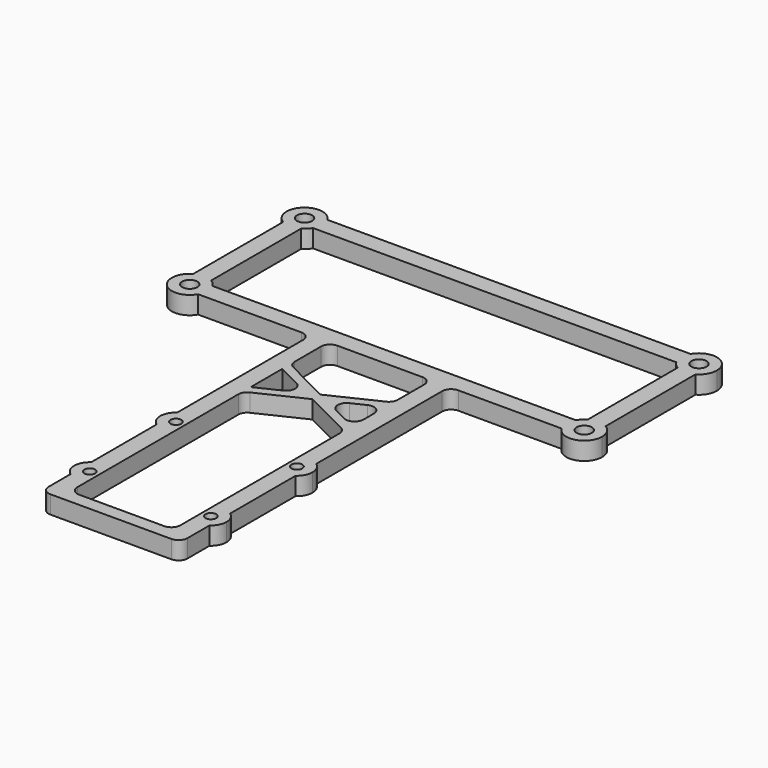
from build123d import *

# Parameters (mm, degrees)
F0_R     = 0.6
F0_R_2   = 0.85
F1_DEPTH = 2
F2_R     = 1


# Not quite as in the source:
# - a feature names something its author has since deleted; it is built from what else it names


with BuildPart() as f1:
    # F0 (on Top) → F1 (new body)
    with BuildSketch(Plane.XY):
        with BuildLine():
            ThreePointArc((-5.75, -27.5638593384), (-6.75, -27.25), (-7.75, -27.5638593384))
            Line((-7.75, -27.5638593384), (-7.75, -30.4361406616))
            ThreePointArc((-7.75, -30.4361406616), (-6.75, -30.75), (-5.75, -30.4361406616))
            Line((-5.75, -30.4361406616), (-5.75, -27.5638593384))
        make_face()
        with Locations((-6.75, -29)):
            Circle(F0_R, mode=Mode.SUBTRACT)
        with BuildLine():
            Line((-7.75, -30.4361406616), (-7.75, -27.5638593384))
            ThreePointArc((-7.75, -27.5638593384), (-8.5, -29), (-7.75, -30.4361406616))
        make_face()
        with BuildLine():
            ThreePointArc((-5.75, -30.4361406616), (-6.75, -30.75), (-7.75, -30.4361406616))
            Line((-7.75, -30.4361406616), (-7.75, -39.5638593384))
            ThreePointArc((-7.75, -39.5638593384), (-6.75, -39.25), (-5.75, -39.5638593384))
            Line((-5.75, -39.5638593384), (-5.75, -30.4361406616))
        make_face()
        with BuildLine():
            Line((-7.75, -42.4361406616), (-7.75, -39.5638593384))
            ThreePointArc((-7.75, -39.5638593384), (-8.5, -41), (-7.75, -42.4361406616))
        make_face()
        with BuildLine():
            ThreePointArc((-5.75, -39.5638593384), (-6.75, -39.25), (-7.75, -39.5638593384))
            Line((-7.75, -39.5638593384), (-7.75, -42.4361406616))
            ThreePointArc((-7.75, -42.4361406616), (-6.75, -42.75), (-5.75, -42.4361406616))
            Line((-5.75, -42.4361406616), (-5.75, -39.5638593384))
        make_face()
        with Locations((-6.75, -41)):
            Circle(F0_R, mode=Mode.SUBTRACT)
        with BuildLine():
            ThreePointArc((-5.75, -42.4361406616), (-6.75, -42.75), (-7.75, -42.4361406616))
            Line((-7.75, -42.4361406616), (-7.75, -46.5))
            Line((-7.75, -46.5), (7.75, -46.5))
            Line((7.75, -46.5), (7.75, -42.4361406616))
            ThreePointArc((7.75, -42.4361406616), (6.75, -42.75), (5.75, -42.4361406616))
            Line((5.75, -42.4361406616), (5.75, -45))
            Line((5.75, -45), (-5.75, -45))
            Line((-5.75, -45), (-5.75, -42.4361406616))
        make_face()
        with BuildLine():
            Line((7.75, -30.4361406616), (7.75, -27.5638593384))
            ThreePointArc((7.75, -27.5638593384), (6.75, -27.25), (5.75, -27.5638593384))
            Line((5.75, -27.5638593384), (5.75, -30.4361406616))
            ThreePointArc((5.75, -30.4361406616), (6.75, -30.75), (7.75, -30.4361406616))
        make_face()
        with Locations((6.75, -29)):
            Circle(F0_R, mode=Mode.SUBTRACT)
        with BuildLine():
            ThreePointArc((8.5, -29), (8.3012092057, -28.1899074127), (7.75, -27.5638593384))
            Line((7.75, -27.5638593384), (7.75, -30.4361406616))
            ThreePointArc((7.75, -30.4361406616), (8.3012092057, -29.8100925873), (8.5, -29))
        make_face()
        with BuildLine():
            Line((7.75, -39.5638593384), (7.75, -30.4361406616))
            ThreePointArc((7.75, -30.4361406616), (6.75, -30.75), (5.75, -30.4361406616))
            Line((5.75, -30.4361406616), (5.75, -39.5638593384))
            ThreePointArc((5.75, -39.5638593384), (6.75, -39.25), (7.75, -39.5638593384))
        make_face()
        with BuildLine():
            Line((7.75, -42.4361406616), (7.75, -39.5638593384))
            ThreePointArc((7.75, -39.5638593384), (6.75, -39.25), (5.75, -39.5638593384))
            Line((5.75, -39.5638593384), (5.75, -42.4361406616))
            ThreePointArc((5.75, -42.4361406616), (6.75, -42.75), (7.75, -42.4361406616))
        make_face()
        with Locations((6.75, -41)):
            Circle(F0_R, mode=Mode.SUBTRACT)
        with BuildLine():
            ThreePointArc((8.5, -41), (8.3012092057, -40.1899074127), (7.75, -39.5638593384))
            Line((7.75, -39.5638593384), (7.75, -42.4361406616))
            ThreePointArc((7.75, -42.4361406616), (8.3012092057, -41.8100925873), (8.5, -41))
        make_face()
        with BuildLine():
            ThreePointArc((-20, -8), (-20.0681483474, -8.5176380902), (-20.2679491924, -9))
            Line((-20.2679491924, -9), (-7.75, -9))
            Line((-7.75, -9), (-5.75, -9))
            Line((-5.75, -9), (5.75, -9))
            Line((5.75, -9), (7.75, -9))
            Line((7.75, -9), (20.2679491924, -9))
            ThreePointArc((20.2679491924, -9), (20, -8), (20.2679491924, -7))
            Line((20.2679491924, -7), (-20.2679491924, -7))
            ThreePointArc((-20.2679491924, -7), (-20.0681483474, -7.4823619098), (-20, -8))
        make_face()
        with BuildLine():
            ThreePointArc((24, -8), (23.7320508076, -7), (23, -6.2679491924))
            Line((23, -6.2679491924), (23, -9))
            Line((23, -9), (20.2679491924, -9))
            ThreePointArc((20.2679491924, -9), (22.5176380902, -9.9318516526), (24, -8))
        make_face()
        with BuildLine():
            ThreePointArc((23, -6.2679491924), (22, -6), (21, -6.2679491924))
            Line((21, -6.2679491924), (21, -7))
            Line((21, -7), (20.2679491924, -7))
            ThreePointArc((20.2679491924, -7), (20, -8), (20.2679491924, -9))
            Line((20.2679491924, -9), (23, -9))
            Line((23, -9), (23, -6.2679491924))
        make_face()
        with Locations((22, -8)):
            Circle(F0_R_2, mode=Mode.SUBTRACT)
        with BuildLine():
            ThreePointArc((23, 6.2679491924), (22, 6), (21, 6.2679491924))
            Line((21, 6.2679491924), (21, -6.2679491924))
            ThreePointArc((21, -6.2679491924), (22, -6), (23, -6.2679491924))
            Line((23, -6.2679491924), (23, 6.2679491924))
        make_face()
        with BuildLine():
            Line((21, -7), (21, -6.2679491924))
            ThreePointArc((21, -6.2679491924), (20.5857864376, -6.5857864376), (20.2679491924, -7))
            Line((20.2679491924, -7), (21, -7))
        make_face()
        with BuildLine():
            Line((21, 7), (20.2679491924, 7))
            ThreePointArc((20.2679491924, 7), (20.5857864376, 6.5857864376), (21, 6.2679491924))
            Line((21, 6.2679491924), (21, 7))
        make_face()
        with BuildLine():
            Line((23, 9), (20.2679491924, 9))
            ThreePointArc((20.2679491924, 9), (20, 8), (20.2679491924, 7))
            Line((20.2679491924, 7), (21, 7))
            Line((21, 7), (21, 6.2679491924))
            ThreePointArc((21, 6.2679491924), (22, 6), (23, 6.2679491924))
            Line((23, 6.2679491924), (23, 9))
        make_face()
        with Locations((22, 8)):
            Circle(F0_R_2, mode=Mode.SUBTRACT)
        with BuildLine():
            ThreePointArc((24, 8), (22.5176380902, 9.9318516526), (20.2679491924, 9))
            Line((20.2679491924, 9), (23, 9))
            Line((23, 9), (23, 6.2679491924))
            ThreePointArc((23, 6.2679491924), (23.7320508076, 7), (24, 8))
        make_face()
        with BuildLine():
            ThreePointArc((-20.2679491924, 9), (-20.0681483474, 8.5176380902), (-20, 8))
            ThreePointArc((-20, 8), (-20.0681483474, 7.4823619098), (-20.2679491924, 7))
            Line((-20.2679491924, 7), (20.2679491924, 7))
            ThreePointArc((20.2679491924, 7), (20, 8), (20.2679491924, 9))
            Line((20.2679491924, 9), (-20.2679491924, 9))
        make_face()
        with BuildLine():
            ThreePointArc((-21, -6.2679491924), (-22, -6), (-23, -6.2679491924))
            Line((-23, -6.2679491924), (-23, -9))
            Line((-23, -9), (-20.2679491924, -9))
            ThreePointArc((-20.2679491924, -9), (-20.0681483474, -8.5176380902), (-20, -8))
            ThreePointArc((-20, -8), (-20.0681483474, -7.4823619098), (-20.2679491924, -7))
            Line((-20.2679491924, -7), (-21, -7))
            Line((-21, -7), (-21, -6.2679491924))
        make_face()
        with Locations((-22, -8)):
            Circle(F0_R_2, mode=Mode.SUBTRACT)
        with BuildLine():
            Line((-23, -9), (-23, -6.2679491924))
            ThreePointArc((-23, -6.2679491924), (-23.4142135624, -9.4142135624), (-20.2679491924, -9))
            Line((-20.2679491924, -9), (-23, -9))
        make_face()
        with BuildLine():
            ThreePointArc((-20.2679491924, -7), (-20.5857864376, -6.5857864376), (-21, -6.2679491924))
            Line((-21, -6.2679491924), (-21, -7))
            Line((-21, -7), (-20.2679491924, -7))
        make_face()
        with BuildLine():
            Line((-23, 9), (-20.2679491924, 9))
            ThreePointArc((-20.2679491924, 9), (-23.4142135624, 9.4142135624), (-23, 6.2679491924))
            Line((-23, 6.2679491924), (-23, 9))
        make_face()
        with BuildLine():
            ThreePointArc((-20.2679491924, 7), (-20.0681483474, 7.4823619098), (-20, 8))
            ThreePointArc((-20, 8), (-20.0681483474, 8.5176380902), (-20.2679491924, 9))
            Line((-20.2679491924, 9), (-23, 9))
            Line((-23, 9), (-23, 6.2679491924))
            ThreePointArc((-23, 6.2679491924), (-22, 6), (-21, 6.2679491924))
            Line((-21, 6.2679491924), (-21, 7))
            Line((-21, 7), (-20.2679491924, 7))
        make_face()
        with Locations((-22, 8)):
            Circle(F0_R_2, mode=Mode.SUBTRACT)
        with BuildLine():
            ThreePointArc((-21, 6.2679491924), (-20.5857864376, 6.5857864376), (-20.2679491924, 7))
            Line((-20.2679491924, 7), (-21, 7))
            Line((-21, 7), (-21, 6.2679491924))
        make_face()
        with BuildLine():
            ThreePointArc((-21, 6.2679491924), (-22, 6), (-23, 6.2679491924))
            Line((-23, 6.2679491924), (-23, -6.2679491924))
            ThreePointArc((-23, -6.2679491924), (-22, -6), (-21, -6.2679491924))
            Line((-21, -6.2679491924), (-21, 6.2679491924))
        make_face()
        with BuildLine():
            Line((7.75, -9), (5.75, -9))
            Line((5.75, -9), (5.75, -14.3142581873))
            Line((5.75, -14.3142581873), (5.75, -15.422623174))
            Line((5.75, -15.422623174), (5.75, -20.073895466))
            Line((5.75, -20.073895466), (5.75, -21.1929723705))
            Line((5.75, -21.1929723705), (5.75, -27.5638593384))
            ThreePointArc((5.75, -27.5638593384), (6.75, -27.25), (7.75, -27.5638593384))
            Line((7.75, -27.5638593384), (7.75, -9))
        make_face()
        Polygon((5.75, -20.073895466), (1.0053343494, -17.6905184824), (-0.1362126115, -18.2361647275), (5.75, -21.1929723705), align=None)
        Polygon((5.75, -15.422623174), (5.75, -14.3142581873), (-0.125285608, -17.1225767595), (1.0053343494, -17.6905184824), align=None)
        Polygon((1.0053343494, -17.6905184824), (-0.125285608, -17.1225767595), (-1.2668325689, -17.6682230047), (-0.1362126115, -18.2361647275), align=None)
        Polygon((-5.75, -19.8111251883), (-5.75, -20.9194901751), (-0.1362126115, -18.2361647275), (-1.2668325689, -17.6682230047), align=None)
        Polygon((-0.125285608, -17.1225767595), (-5.75, -14.2971269157), (-5.75, -15.4162038202), (-1.2668325689, -17.6682230047), align=None)
        with BuildLine():
            Line((-5.75, -9), (-7.75, -9))
            Line((-7.75, -9), (-7.75, -27.5638593384))
            ThreePointArc((-7.75, -27.5638593384), (-6.75, -27.25), (-5.75, -27.5638593384))
            Line((-5.75, -27.5638593384), (-5.75, -20.9194901751))
            Line((-5.75, -20.9194901751), (-5.75, -19.8111251883))
            Line((-5.75, -19.8111251883), (-5.75, -15.4162038202))
            Line((-5.75, -15.4162038202), (-5.75, -14.2971269157))
            Line((-5.75, -14.2971269157), (-5.75, -9))
        make_face()
    extrude(amount=F1_DEPTH)

    # F2
    f2_edges = [f1.edges().sort_by_distance(p)[0] for p in [
        (-7.75, -46.5, 1),
        (7.75, -46.5, 1),
        (-5.75, -45, 1),
        (5.75, -45, 1),
        (-5.75, -20.91949, 1),
        (5.75, -21.192972, 1),
        (5.75, -20.073895, 1),
        (5.75, -15.422623, 1),
        (1.005334, -17.690518, 1),
        (-1.266833, -17.668223, 1),
        (-5.75, -14.297127, 1),
        (5.75, -14.314258, 1),
        (5.75, -9, 1),
        (-5.75, -9, 1),
        (-7.75, -9, 1),
        (7.75, -9, 1),
    ]]
    fillet(f2_edges, radius=F2_R)


solid = f1.part
